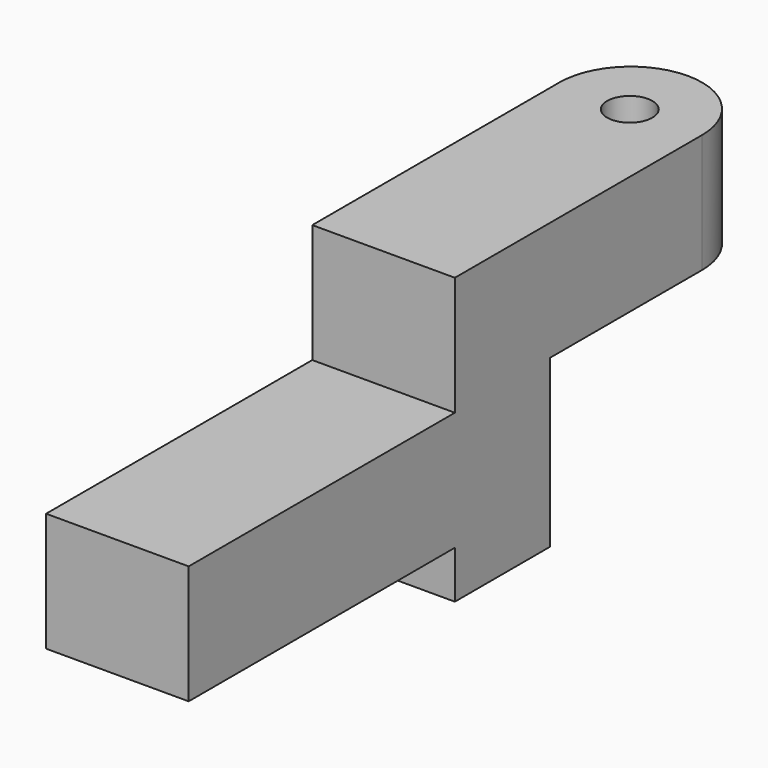
from build123d import *

# Parameters (mm, degrees)
F1_DEPTH = 15
F3_D     = 19.1
F3_DEPTH = 14
F3_TIP   = 5.7382189117
F5_R     = 14.99999
F6_D     = 9.525


# Not quite as in the source:
# - a fillet or chamfer is up to 0.001 mm smaller than in the source, because OpenCascade refuses the exact size
# - a length typed as a fraction of an inch, garbled in the dataset ("3 / 203.2 mm" for 3/8 in), is restored


with BuildPart() as f1:
    # F0 (on Right) → F1 (new body, symmetric)
    with BuildSketch(Plane.YZ):
        Polygon((0, -35), (0, 0), (55, 0), (55, 25), (-25, 25), (-25, 0), (-95, 0), (-95, -25), (-25, -25), (-25, -35), align=None)
    extrude(amount=F1_DEPTH, both=True)

    # F3
    with Locations(Plane(origin=(0, 0, 0), x_dir=(-1, 0, 0), z_dir=(0, 1, 0))):
        with Locations((0, -19.5)):
            Hole(F3_D / 2, depth=F3_DEPTH)
            with Locations((0, 0, -(F3_DEPTH + F3_TIP / 2))):  # 118° drill point
                Cone(0, F3_D / 2, F3_TIP, mode=Mode.SUBTRACT)

    # F5 (radius 15 in the source; OpenCascade refuses exactly that, so slightly less here)
    f5_edges = [f1.edges().sort_by_distance(p)[0] for p in [
        (-15, 55, 12.5),
        (15, 55, 12.5),
    ]]
    fillet(f5_edges, radius=F5_R)

    # F6 (through all)
    with Locations(Plane(origin=(0, 0, 0), x_dir=(1, 0, 0), z_dir=(0, 0, -1))):
        with Locations((0, -39.75)):
            Hole(F6_D / 2)


solid = f1.part
